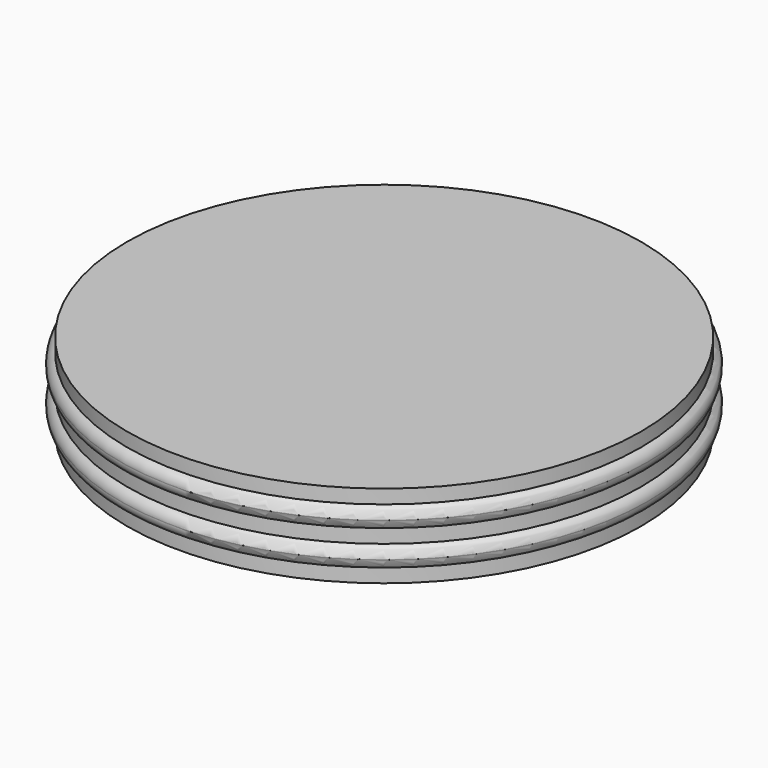
from build123d import *

# Parameters (mm, degrees)
F0_R     = 37
F1_DEPTH = 2
F2_R     = 38
F3_DEPTH = 3
F4_R     = 37
F5_DEPTH = 2
F6_R     = 38
F7_DEPTH = 3
F8_R     = 37
F9_DEPTH = 2


# Not quite as in the source:
# - a fillet or chamfer that OpenCascade refuses, or shapes differently, is made with other operations: its cross-section is extruded or revolved along the edge and cut away or added


with BuildPart() as f1:
    # F0 (on Top) → F1 (new body)
    with BuildSketch(Plane.XY):
        Circle(F0_R)
    extrude(amount=F1_DEPTH)

    # F2 (on face) → F3 (join)
    with BuildSketch(Plane.XY.offset(2)):
        Circle(F2_R)
    extrude(amount=F3_DEPTH)

    # F4 (on face) → F5 (join)
    with BuildSketch(Plane.XY.offset(5)):
        Circle(F4_R)
    extrude(amount=F5_DEPTH)

    # F6 (on face) → F7 (join)
    with BuildSketch(Plane.XY.offset(7)):
        Circle(F6_R)
    extrude(amount=F7_DEPTH)

    # F8 (on face) → F9 (join)
    with BuildSketch(Plane.XY.offset(10)):
        Circle(F8_R)
    extrude(amount=F9_DEPTH)

    # F10: fillet of radius 1.6 on 4 edges, made by hand

    # F10_s1 → F10_t2 (revolve, cut)
    with BuildSketch(Plane.XZ):
        with BuildLine():
            ThreePointArc((38, 8.4832396974), (37.7266499161, 7.5888125064), (37, 7))
            Line((37, 7), (38, 7))
            Line((38, 7), (38, 8.4832396974))
        make_face()
    revolve(axis=Axis((0, 0, 7), (0, 0, 1)), mode=Mode.SUBTRACT)

    # F10_s3 → F10_t4 (revolve, cut)
    with BuildSketch(Plane.XZ):
        with BuildLine():
            ThreePointArc((38, 3.4832396974), (37.7266499161, 2.5888125064), (37, 2))
            Line((37, 2), (38, 2))
            Line((38, 2), (38, 3.4832396974))
        make_face()
    revolve(axis=Axis((0, 0, 2), (0, 0, 1)), mode=Mode.SUBTRACT)

    # F10_s5 → F10_t6 (revolve, cut)
    with BuildSketch(Plane.XZ):
        with BuildLine():
            ThreePointArc((38, 8.5167603026), (37.7266499161, 9.4111874936), (37, 10))
            Line((37, 10), (38, 10))
            Line((38, 10), (38, 8.5167603026))
        make_face()
    revolve(axis=Axis((0, 0, 10), (0, 0, 1)), mode=Mode.SUBTRACT)

    # F10_s7 → F10_t8 (revolve, cut)
    with BuildSketch(Plane.XZ):
        with BuildLine():
            ThreePointArc((37, 5), (37.7266499161, 4.4111874936), (38, 3.5167603026))
            Line((38, 3.5167603026), (38, 5))
            Line((38, 5), (37, 5))
        make_face()
    revolve(axis=Axis((0, 0, 5), (0, 0, 1)), mode=Mode.SUBTRACT)


solid = f1.part
